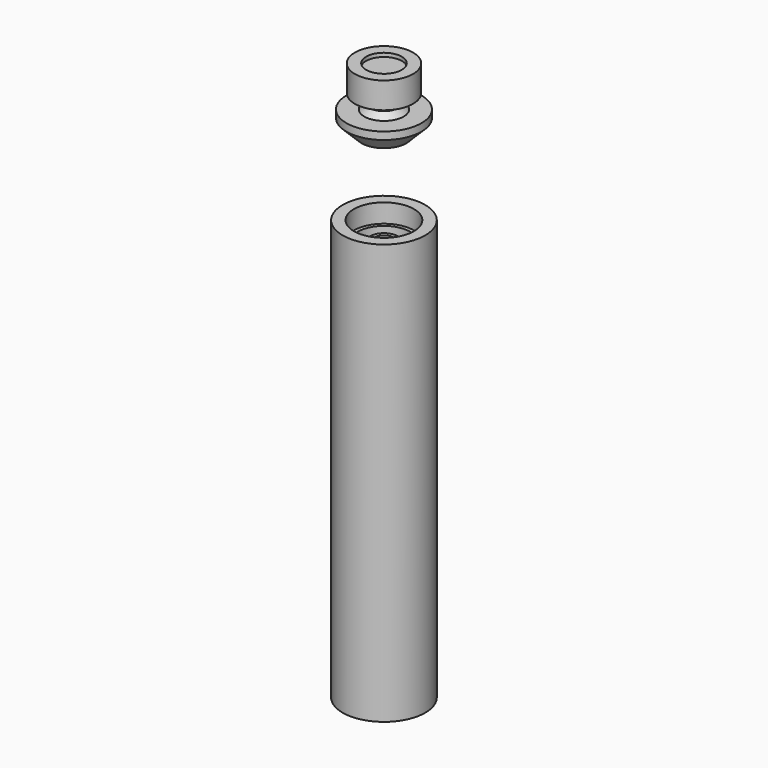
from build123d import *

# Parameters (mm, degrees)
F0_W    = 1
F0_H    = 1.5
F2_W    = 1
F2_H    = 100
F6_SIZE = 1.49999
F7_W    = 3
F7_H    = 1


# Not quite as in the source:
# - a fillet or chamfer is up to 0.001 mm smaller than in the source, because OpenCascade refuses the exact size


with BuildPart() as f1:
    # F0 (on Front) → F1 (revolve)
    with BuildSketch(Plane.XZ):
        Polygon((-6, 0), (-2.75, 0), (-2.75, 6), (-3.75, 6), (-10, 6), (-10, 4), align=None)
        with Locations((-3.25, 6.75)):
            Rectangle(F0_W, F0_H)
    revolve(axis=Axis((0, 0, 7.7176861543), (0, 0, 1)))

    # F6 (size 1.5 in the source; OpenCascade refuses exactly that, so slightly less here)
    f6_edges = [f1.edges().sort_by_distance(p)[0] for p in [
        (3.75, 0, 6),
    ]]
    chamfer(f6_edges, length=F6_SIZE)


with BuildPart() as f3:
    # F2 (on Front) → F3 (revolve)
    with BuildSketch(Plane.XZ):
        with Locations((-3.25, -75)):
            Rectangle(F2_W, F2_H)
        Polygon((-4.75, -124), (-3.75, -125), (-3.75, -25), (-4.75, -26), align=None)
    revolve(axis=Axis((0, 0, -10.3056698131), (0, 0, -1)))


with BuildPart() as f5:
    # F4 (on Front) → F5 (revolve)
    with BuildSketch(Plane.XZ):
        Polygon((-8, -20), (-11, -20), (-11, -132), (-8.5, -132), (-8.5, -122), (-7, -120.5), (-7, -25), (-8, -25), align=None)
    revolve(axis=Axis((0, 0, -133.877441287), (0, 0, -1)))


with BuildPart() as f8:
    # F7 (on Front) → F8 (revolve)
    with BuildSketch(Plane.XZ):
        with Locations((-6.25, 16.3010139478)):
            Rectangle(F7_W, F7_H)
        Polygon((-7.75, 9.8010139478), (0, 9.8010139478), (0, 15.8010139478), (-4.75, 15.8010139478), (-7.75, 15.8010139478), align=None)
    revolve(axis=Axis((0, 0, 9.0013529551), (0, 0, 1)))


solid = Compound([f1.part, f3.part, f5.part, f8.part])
